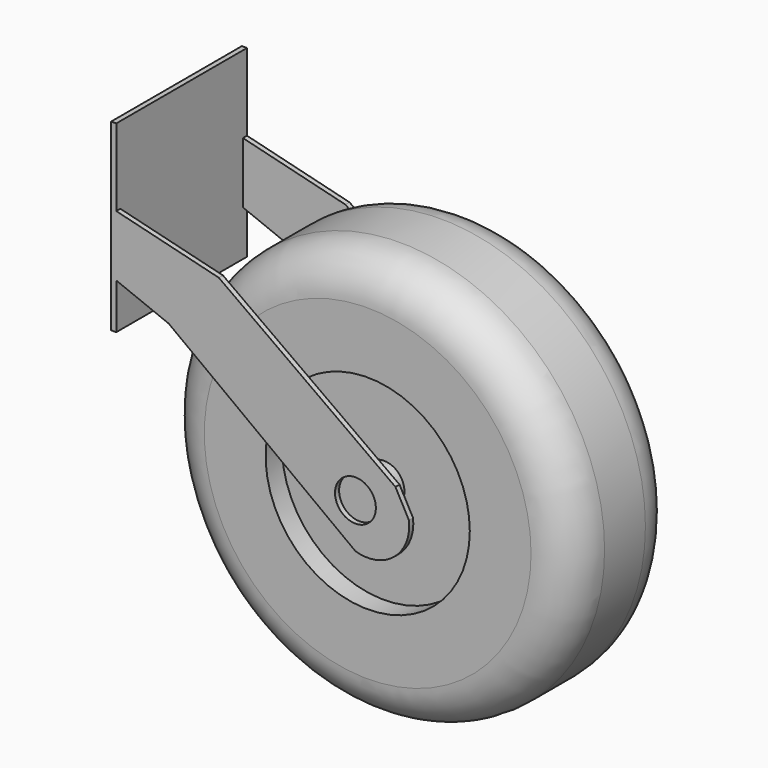
from build123d import *

# Parameters (mm, degrees)
F0_R      = 127
F1_DEPTH  = 82.55
F2_R      = 25.4
F3_R      = 63.5
F4_DEPTH  = 12.7
F5_R      = 63.5
F7_DEPTH  = 12.7
F8_R      = 12.7
F9_DEPTH  = 19.05
F10_R     = 12.7
F11_DEPTH = 19.05
F12_R     = 12.7
F13_DEPTH = 3.175
F15_W     = 3.175
F15_H     = 37.9564044358
F16_DEPTH = 3.175


# Not quite as in the source:
# - a length typed as a fraction of an inch, garbled in the dataset ("3 / 203.2 mm" for 3/8 in), is restored


with BuildPart() as f1:
    # F0 (on Front) → F1 (new body)
    with BuildSketch(Plane.XZ):
        Circle(F0_R)
    extrude(amount=F1_DEPTH)

    # F2
    f2_edges = [f1.edges().sort_by_distance(p)[0] for p in [
        (-127, 0, 0),
        (-127, -82.55, 0),
    ]]
    fillet(f2_edges, radius=F2_R)

    # F3 (on face) → F4 (cut)
    with BuildSketch(Plane.XZ.offset(82.55)):
        Circle(F3_R)
    extrude(amount=-F4_DEPTH, mode=Mode.SUBTRACT)

    # F5 (on face) → F7 (cut)
    with BuildSketch(Plane(origin=(0, 0, 0), x_dir=(-1, 0, 0), z_dir=(0, 1, 0))):
        Circle(F5_R)
    extrude(amount=-F7_DEPTH, mode=Mode.SUBTRACT)

    # F8 (on face) → F9 (join)
    with BuildSketch(Plane(origin=(0, -12.7, 0), x_dir=(-1, 0, 0), z_dir=(0, 1, 0))):
        Circle(F8_R)
    extrude(amount=F9_DEPTH)

    # F10 (on face) → F11 (join)
    with BuildSketch(Plane.XZ.offset(69.85)):
        Circle(F10_R)
    extrude(amount=F11_DEPTH)


with BuildPart() as f13:
    # F12 (on face) → F13 (new body)
    with BuildSketch(Plane.XZ.offset(88.9)):
        with BuildLine():
            Line((-116.1441206932, 59.0758956969), (0, -27.7741849422))
            ThreePointArc((0, -27.7741849422), (24.1842527019, -22.9319763652), (33.2644246519, 0))
            Line((33.2644246519, 0), (24.8675793409, 15.5018689111))
            Line((24.8675793409, 15.5018689111), (-84.9373340607, 94.303034246))
            Line((-84.9373340607, 94.303034246), (-148.7210690975, 110.0305374596))
            Line((-148.7210690975, 110.0305374596), (-148.7210690975, 72.0741330239))
            Line((-148.7210690975, 72.0741330239), (-116.1441206932, 59.0758956969))
        make_face()
        Circle(F12_R, mode=Mode.SUBTRACT)
    extrude(amount=F13_DEPTH)


with BuildPart() as f14_1:
    # F14: instance of F13
    add(f13.part.mirror(Plane.XZ.offset(41.275)))


with BuildPart() as f13_1:
    add(f13.part)

    # F15 (on face) → F16 (join)
    with BuildSketch(Plane(origin=(-148.7210690975, 0, 0), x_dir=(0, -1, 0), z_dir=(-1, 0, 0))):
        Polygon((-9.525, 72.0741330239), (-9.525, 43.7358616628), (92.075, 43.7358616628), (92.075, 158.0358616628), (-9.525, 158.0358616628), (-9.525, 110.0305374596), (-6.35, 110.0305374596), (-6.35, 72.0741330239), align=None)
        with Locations((-7.9375, 91.0523352418)):
            Rectangle(F15_W, F15_H)
    extrude(amount=F16_DEPTH)


solid = Compound([f1.part, f14_1.part, f13_1.part])
